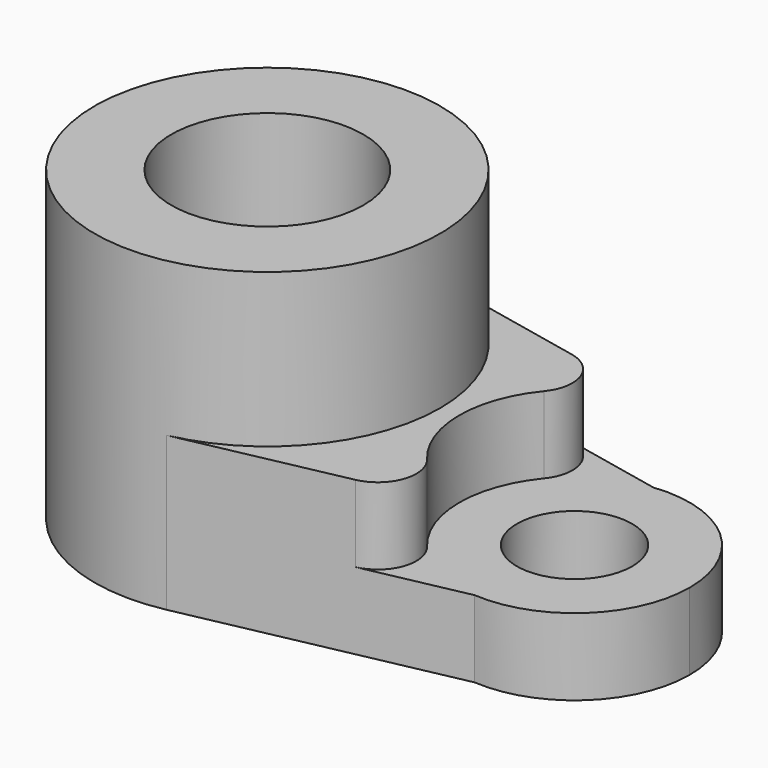
from build123d import *

# Parameters (mm, degrees)
F0_R     = 15.875
F1_DEPTH = 50.8
F2_DEPTH = 25.4
F0_R_2   = 9.525
F3_DEPTH = 12.7
F4_R     = 6.35


with BuildPart() as f1:
    # F0 (on Top) → F1 (new body)
    with BuildSketch(Plane.XY):
        with BuildLine():
            ThreePointArc((4.8347544076, 0), (-1.5460097383, 17.998514379), (-17.8386678043, 27.9589342538))
            ThreePointArc((-17.8386678043, 27.9589342538), (-52.3151461351, 0.07539214), (-17.9862828844, -27.9896862818))
            ThreePointArc((-17.9862828844, -27.9896862818), (-1.5935741791, -18.0570088971), (4.8347544076, 0))
        make_face()
        with Locations((-23.7402455924, 0)):
            Circle(F0_R, mode=Mode.SUBTRACT)
    extrude(amount=F1_DEPTH)

    # F0 (on Top) → F2 (join)
    with BuildSketch(Plane.XY):
        with BuildLine():
            ThreePointArc((25.7271171156, -19.0033307041), (8.0139347128, -0.3990640994), (24.9322885076, 18.9308316998))
            Line((24.9322885076, 18.9308316998), (-17.8386678043, 27.9589342538))
            ThreePointArc((-17.8386678043, 27.9589342538), (-1.5460097383, 17.998514379), (4.8347544076, 0))
            ThreePointArc((4.8347544076, 0), (-1.5935741791, -18.0570088971), (-17.9862828844, -27.9896862818))
            Line((-17.9862828844, -27.9896862818), (25.7271171156, -19.0033307041))
        make_face()
    extrude(amount=F2_DEPTH)

    # F0 (on Top) → F3 (join)
    with BuildSketch(Plane.XY):
        with BuildLine():
            ThreePointArc((25.7271171156, -19.0033307041), (40.0504387542, -13.9335788729), (46.1097544076, 0))
            ThreePointArc((46.1097544076, 0), (39.7557040492, 14.2026533682), (24.9322885076, 18.9308316998))
            ThreePointArc((24.9322885076, 18.9308316998), (8.0139347128, -0.3990640994), (25.7271171156, -19.0033307041))
        make_face()
        with Locations((27.0597544076, 0)):
            Circle(F0_R_2, mode=Mode.SUBTRACT)
    extrude(amount=F3_DEPTH)

    # F4
    f4_edges = [f1.edges().sort_by_distance(p)[0] for p in [
        (25.727117, -19.003331, 19.05),
        (24.932289, 18.930832, 19.05),
    ]]
    fillet(f4_edges, radius=F4_R)


solid = f1.part
